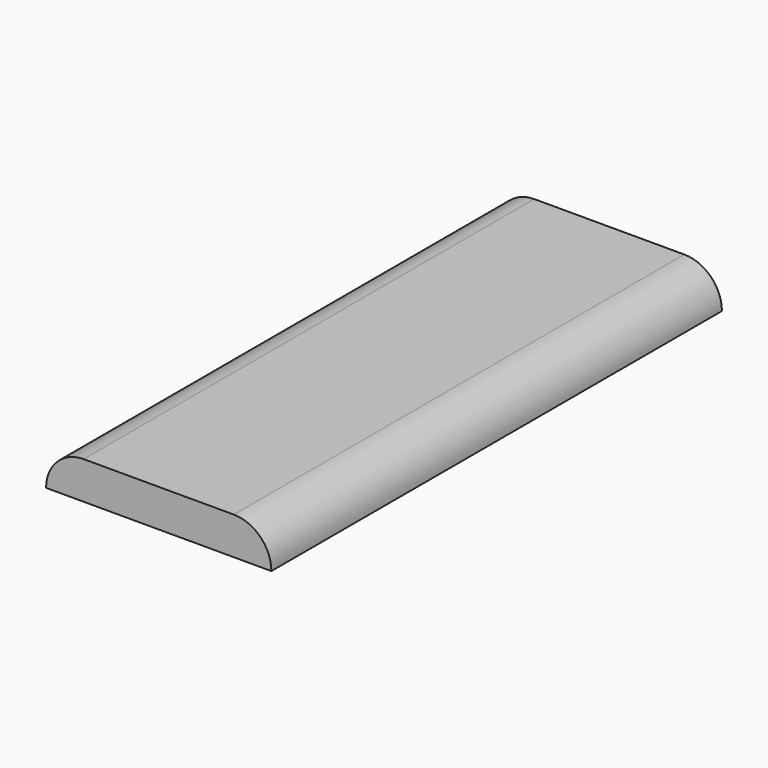
from build123d import *

# Parameters (mm, degrees)
F0_W     = 30
F0_H     = 75
F1_DEPTH = 2.5
F2_R     = 4.99999


# Not quite as in the source:
# - a fillet or chamfer is up to 0.001 mm smaller than in the source, because OpenCascade refuses the exact size


with BuildPart() as f1:
    # F0 (on Top) → F1 (new body, symmetric)
    with BuildSketch(Plane.XY):
        Rectangle(F0_W, F0_H)
    extrude(amount=F1_DEPTH, both=True)

    # F2 (radius 5 in the source; OpenCascade refuses exactly that, so slightly less here)
    f2_edges = [f1.edges().sort_by_distance(p)[0] for p in [
        (15, 0, 2.5),
        (-15, 0, 2.5),
    ]]
    fillet(f2_edges, radius=F2_R)


solid = f1.part
